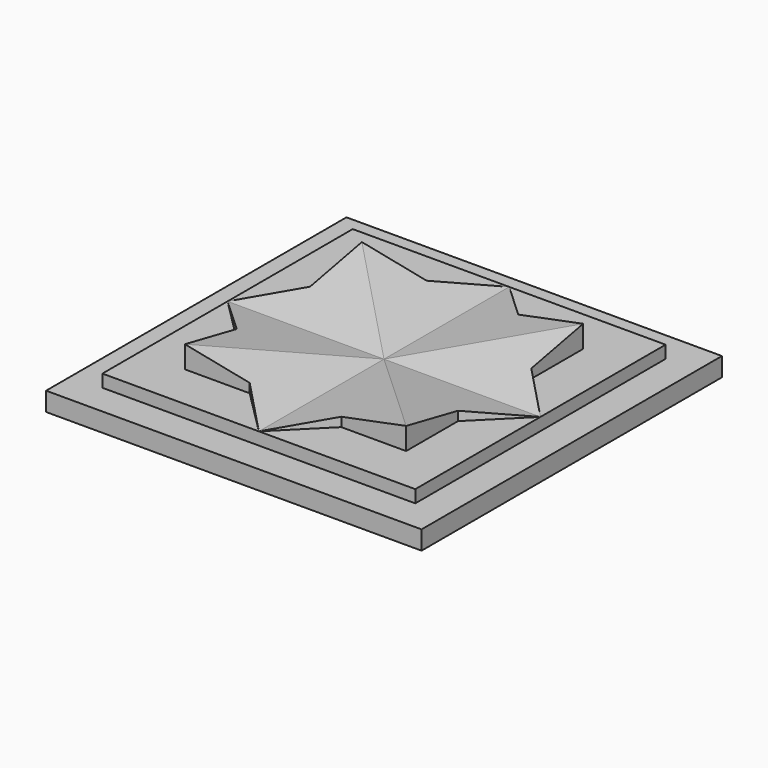
from build123d import *

# Parameters (mm, degrees)
F1_DEPTH = 10
F2_SIZE2 = 24.99999
F2_SIZE  = 4.99999
F4_COUNT = 4
F5_W     = 60
F5_H     = 60
F5_W_2   = 50
F5_H_2   = 50
F6_DEPTH = 15
F8_DEPTH = 10
F9_DEPTH = 12


# Not quite as in the source:
# - a fillet or chamfer is up to 0.001 mm smaller than in the source, because OpenCascade refuses the exact size


with BuildPart() as f1:
    # F0 (on Top) → F1 (new body)
    with BuildSketch(Plane.XY):
        Polygon((-25, 0), (0, 0), (-25, 25), align=None)
        Polygon((-25, 25), (0, 0), (0, 25), align=None)
    extrude(amount=F1_DEPTH)

    # F2 (size 5 and 25 in the source; OpenCascade refuses exactly that, so slightly less here)
    f2_edges = [f1.edges().sort_by_distance(p)[0] for p in [
        (-12.5, 0, 10),
        (0, 12.5, 10),
    ]]
    chamfer(f2_edges, length=F2_SIZE, length2=F2_SIZE2)


with BuildPart() as f4_1:
    # F4: instance of F1
    add(f1.part.rotate(Axis((0, 0, -0.4458203912), (0, 0, -1)), 1 * 360 / F4_COUNT))


with BuildPart() as f4_2:
    # F4: instance of F1
    add(f1.part.rotate(Axis((0, 0, -0.4458203912), (0, 0, -1)), 2 * 360 / F4_COUNT))


with BuildPart() as f4_3:
    # F4: instance of F1
    add(f1.part.rotate(Axis((0, 0, -0.4458203912), (0, 0, -1)), 3 * 360 / F4_COUNT))


with BuildPart() as f1_1:
    add(f1.part)

    add(f4_1.part)  # F6 merges F4_1

    add(f4_2.part)  # F6 merges F4_2

    add(f4_3.part)  # F6 merges F4_3
    # F5 (on face) → F6 (join)
    with BuildSketch(Plane(origin=(0, 0, 0), x_dir=(1, 0, 0), z_dir=(0, 0, -1))):
        Rectangle(F5_W, F5_H)
        Rectangle(F5_W_2, F5_H_2, mode=Mode.SUBTRACT)
    extrude(amount=-F6_DEPTH)

    # F7 (on face) → F8 (cut)
    with BuildSketch(Plane.XY.offset(15)):
        Polygon((25, 25), (0, 25), (7.3223304703, 17.6776695297), (17.6776695297, 17.6776695297), (17.6776695297, 7.3223304703), (25, 0), align=None)
        Polygon((-7.3223304703, 17.6776695297), (0, 25), (-25, 25), (-25, 0), (-17.6776695297, 7.3223304703), (-17.6776695297, 17.6776695297), align=None)
        Polygon((-17.6776695297, -7.3223304703), (-25, 0), (-25, -25), (0, -25), (-7.3223304703, -17.6776695297), (-17.6776695297, -17.6776695297), align=None)
        Polygon((25, -25), (25, 0), (17.6776695297, -7.3223304703), (17.6776695297, -17.6776695297), (7.3223304703, -17.6776695297), (0, -25), align=None)
    extrude(amount=-F8_DEPTH, mode=Mode.SUBTRACT)

    # F9 (cut): a face of the model
    f9_faces = [f1_1.faces().sort_by_distance(p)[0] for p in [
        (0, 29.1514718626, 15),
    ]]
    extrude(f9_faces, amount=-F9_DEPTH, mode=Mode.SUBTRACT)


solid = f1_1.part
